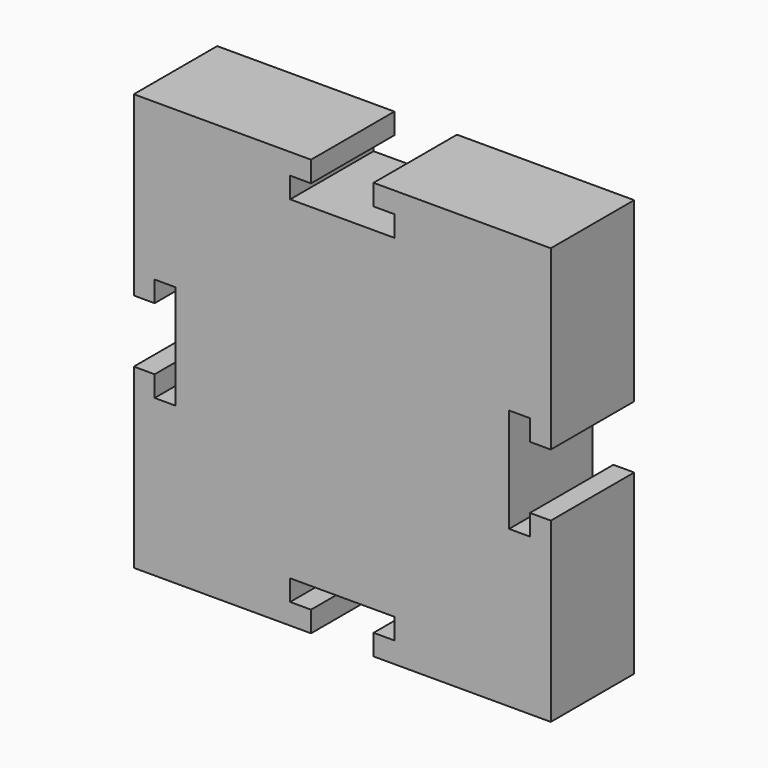
from build123d import *

# Parameters (mm, degrees)
F0_W            = 100
F0_H            = 100
F2_DEPTH        = 25
F4_DEPTH        = 25.001
F4_COPIES_COUNT = 4


# Not quite as in the source:
# - a pattern or mirror of a feature is missing from the dataset's text; its kind, count and spacing are read off the source's solid


with BuildPart() as f2:
    # F0 (on Front) → F2 (new body)
    with BuildSketch(Plane.XZ):
        Rectangle(F0_W, F0_H)
    extrude(amount=F2_DEPTH)

    # F3 (on Front) → F4 (cut, through all)
    with BuildSketch(Plane.XZ):
        Polygon((7.5, 50), (0, 50), (-7.5, 50), (-7.5, 45), (-12.5, 45), (-12.5, 40), (0, 40), (12.5, 40), (12.5, 45), (7.5, 45), align=None)
    f4 = extrude(amount=F4_DEPTH, mode=Mode.SUBTRACT)

    # F4_copies: F4 ×4 about axis
    f4_copies_axis = Axis((0, 0, 0), (0, 1, 0))
    for i in range(1, F4_COPIES_COUNT):
        add(f4.rotate(f4_copies_axis, i * 360 / F4_COPIES_COUNT), mode=Mode.SUBTRACT)


solid = f2.part
